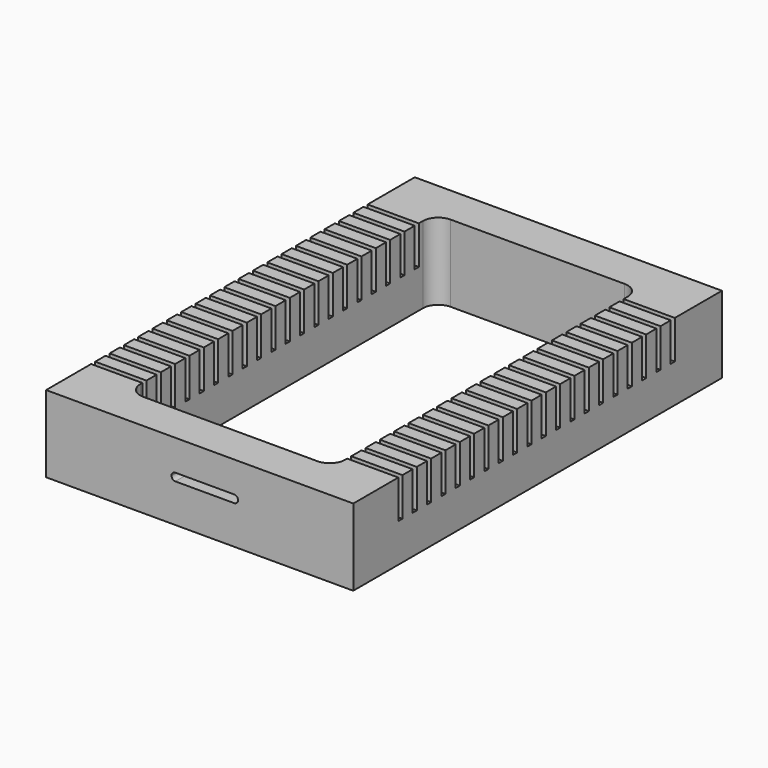
from build123d import *

# Parameters (mm, degrees)
F0_W     = 60
F0_H     = 90
F1_DEPTH = 15
F2_W     = 60
F2_H     = 1
F3_DEPTH = 7.5
F4_W     = 13
F4_H     = 1.5
F5_DEPTH = 3
F6_R     = 0.74999
F7_W     = 13
F7_H     = 1.5
F8_DEPTH = 3
F9_R     = 0.74999


# Not quite as in the source:
# - a fillet or chamfer is up to 0.001 mm smaller than in the source, because OpenCascade refuses the exact size


with BuildPart() as f1:
    # F0 (on Top) → F1 (new body)
    with BuildSketch(Plane.XY):
        Rectangle(F0_W, F0_H)
        with BuildLine():
            ThreePointArc((-20, 34.5), (-19.1213203436, 36.6213203436), (-17, 37.5))
            Line((-17, 37.5), (17, 37.5))
            ThreePointArc((17, 37.5), (19.1213203436, 36.6213203436), (20, 34.5))
            Line((20, 34.5), (20, -34.5))
            ThreePointArc((20, -34.5), (19.1213203436, -36.6213203436), (17, -37.5))
            Line((17, -37.5), (-17, -37.5))
            ThreePointArc((-17, -37.5), (-19.1213203436, -36.6213203436), (-20, -34.5))
            Line((-20, -34.5), (-20, 34.5))
        make_face(mode=Mode.SUBTRACT)
    extrude(amount=F1_DEPTH)

    # F2 (on face) → F3 (cut)
    with BuildSketch(Plane.XY.offset(15)):
        with Locations((0, -33.5)):
            Rectangle(F2_W, F2_H)
        with Locations((0, -30)):
            Rectangle(F2_W, F2_H)
        with Locations((0, -26.5)):
            Rectangle(F2_W, F2_H)
        with Locations((0, -23)):
            Rectangle(F2_W, F2_H)
        with Locations((0, -19.5)):
            Rectangle(F2_W, F2_H)
        with Locations((0, -16)):
            Rectangle(F2_W, F2_H)
        with Locations((0, -12.5)):
            Rectangle(F2_W, F2_H)
        with Locations((0, -9)):
            Rectangle(F2_W, F2_H)
        with Locations((0, -5.5)):
            Rectangle(F2_W, F2_H)
        with Locations((0, -2)):
            Rectangle(F2_W, F2_H)
        with Locations((0, 1.5)):
            Rectangle(F2_W, F2_H)
        with Locations((0, 5)):
            Rectangle(F2_W, F2_H)
        with Locations((0, 8.5)):
            Rectangle(F2_W, F2_H)
        with Locations((0, 12)):
            Rectangle(F2_W, F2_H)
        with Locations((0, 15.5)):
            Rectangle(F2_W, F2_H)
        with Locations((0, 19)):
            Rectangle(F2_W, F2_H)
        with Locations((0, 22.5)):
            Rectangle(F2_W, F2_H)
        with Locations((0, 26)):
            Rectangle(F2_W, F2_H)
        with Locations((0, 29.5)):
            Rectangle(F2_W, F2_H)
        with Locations((0, 33)):
            Rectangle(F2_W, F2_H)
    extrude(amount=-F3_DEPTH, mode=Mode.SUBTRACT)

    # F4 (on face) → F5 (cut)
    with BuildSketch(Plane.XZ.offset(45)):
        with Locations((1, 8.25)):
            Rectangle(F4_W, F4_H)
    extrude(amount=-F5_DEPTH, mode=Mode.SUBTRACT)

    # F6 (radius 0.75 in the source; OpenCascade refuses exactly that, so slightly less here)
    f6_edges = [f1.edges().sort_by_distance(p)[0] for p in [
        (-5.5, -43.5, 7.5),
        (-5.5, -43.5, 9),
        (7.5, -43.5, 7.5),
        (7.5, -43.5, 9),
    ]]
    fillet(f6_edges, radius=F6_R)

    # F7 (on face) → F8 (cut)
    with BuildSketch(Plane(origin=(0, 45, 0), x_dir=(-1, 0, 0), z_dir=(0, 1, 0))):
        with Locations((-1, 8.25)):
            Rectangle(F7_W, F7_H)
    extrude(amount=-F8_DEPTH, mode=Mode.SUBTRACT)

    # F9 (radius 0.75 in the source; OpenCascade refuses exactly that, so slightly less here)
    f9_edges = [f1.edges().sort_by_distance(p)[0] for p in [
        (-5.5, 43.5, 7.5),
        (-5.5, 43.5, 9),
        (7.5, 43.5, 9),
        (7.5, 43.5, 7.5),
    ]]
    fillet(f9_edges, radius=F9_R)


solid = f1.part
